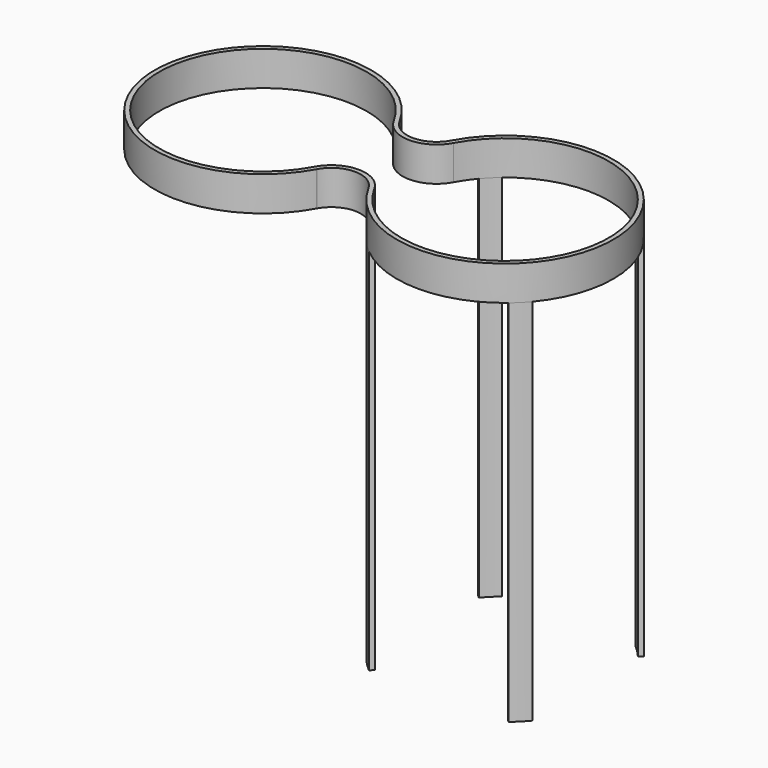
from build123d import *

# Parameters (mm, degrees)
F1_DEPTH = 15
F3_DEPTH = 160


# Not quite as in the source:
# - after a boolean that leaves OpenCascade's solid faulty, fix() repairs it


with BuildPart() as f1:
    # F0 (on Top) → F1 (new body)
    with BuildSketch(Plane.XY):
        with BuildLine():
            ThreePointArc((41.3226906327, -22.3927496943), (52.5, -15.7816452182), (63.6773093673, -22.3927496943))
            ThreePointArc((63.6773093673, -22.3927496943), (63.7058777697, -22.4450182881), (63.7342017495, -22.4974197353))
            ThreePointArc((63.7342017494, -22.4974197352), (152, 0), (63.7342017494, 22.4974197352))
            ThreePointArc((63.7342017494, 22.4974197352), (63.7058777696, 22.445018288), (63.6773093673, 22.3927496943))
            ThreePointArc((63.6773093673, 22.3927496943), (52.5, 15.7816452182), (41.3226906327, 22.3927496943))
            ThreePointArc((41.3226906327, 22.3927496943), (41.2941222304, 22.445018288), (41.2657982506, 22.4974197352))
            ThreePointArc((41.2657982506, 22.4974197352), (-47, 0), (41.2657982506, -22.4974197352))
            ThreePointArc((41.2657982506, -22.4974197352), (41.2941222304, -22.445018288), (41.3226906327, -22.3927496943))
        make_face()
        with BuildLine():
            ThreePointArc((39.5041211148, 21.5505084615), (39.5355894457, 21.4927235868), (39.5669732516, 21.4348927618))
            ThreePointArc((39.5669732516, 21.4348927618), (52.5, 13.7816452182), (65.4330267484, 21.4348927618))
            ThreePointArc((65.4330267484, 21.4348927618), (65.4644105543, 21.4927235868), (65.4958788852, 21.5505084615))
            ThreePointArc((65.4958788852, 21.5505084615), (150, 0), (65.4958788852, -21.5505084615))
            ThreePointArc((65.4958788852, -21.5505084615), (65.4644105543, -21.4927235868), (65.4330267484, -21.4348927618))
            ThreePointArc((65.4330267484, -21.4348927618), (63.4899302841, -18.6916573179), (60.976304449, -16.4594723499))
            ThreePointArc((60.976304449, -16.4594723499), (49.1601952928, -14.1646192224), (39.5669732516, -21.4348927618))
            ThreePointArc((39.5669732516, -21.4348927618), (39.5355894457, -21.4927235868), (39.5041211148, -21.5505084615))
            ThreePointArc((39.5041211148, -21.5505084615), (-45, 0), (39.5041211148, 21.5505084615))
        make_face(mode=Mode.SUBTRACT)
    extrude(amount=F1_DEPTH)

    # F2 (on face) → F3 (join)
    with BuildSketch(Plane(origin=(0, 0, 0), x_dir=(1, 0, 0), z_dir=(0, 0, -1))):
        with BuildLine():
            ThreePointArc((74.7889823447, 36.0040888266), (73.2472602421, 34.6520348301), (71.7659812842, 33.2340187158))
            Line((71.7659812842, 33.2340187158), (73.1801948457, 31.8198051543))
            ThreePointArc((73.1801948466, 31.8198051534), (74.5984406573, 33.1774801565), (76.0745575641, 34.4719999404))
            Line((76.0745575641, 34.4719999404), (74.7889823447, 36.0040888266))
        make_face()
        with BuildLine():
            ThreePointArc((71.7659812842, 33.2340187158), (70.3479651699, 31.7527397579), (68.9959111734, 30.2110176553))
            Line((68.9959111734, 30.2110176553), (70.5280000596, 28.9254424359))
            ThreePointArc((70.5280000596, 28.9254424359), (71.8225198435, 30.4015593427), (73.1801948466, 31.8198051534))
            Line((73.1801948457, 31.8198051543), (71.7659812842, 33.2340187158))
        make_face()
        with BuildLine():
            ThreePointArc((141.0040888266, 30.2110176553), (138.2340187158, 33.2340187158), (135.2110176553, 36.0040888266))
            Line((135.2110176553, 36.0040888266), (133.9254424359, 34.4719999404))
            ThreePointArc((133.9254424359, 34.4719999404), (136.8198051534, 31.8198051534), (139.4719999404, 28.9254424359))
            Line((139.4719999404, 28.9254424359), (141.0040888266, 30.2110176553))
        make_face()
        with BuildLine():
            ThreePointArc((135.2110176553, -36.0040888266), (138.2340187158, -33.2340187158), (141.0040888266, -30.2110176553))
            Line((141.0040888266, -30.2110176553), (139.4719999404, -28.9254424359))
            ThreePointArc((139.4719999404, -28.9254424359), (136.8198051534, -31.8198051534), (133.9254424359, -34.4719999404))
            Line((133.9254424359, -34.4719999404), (135.2110176553, -36.0040888266))
        make_face()
        with BuildLine():
            Line((70.5280000596, -28.9254424359), (68.9959111734, -30.2110176553))
            ThreePointArc((68.9959111734, -30.2110176553), (71.7659812842, -33.2340187158), (74.7889823447, -36.0040888266))
            Line((74.7889823447, -36.0040888266), (76.0745575641, -34.4719999404))
            ThreePointArc((76.0745575641, -34.4719999404), (73.1801948466, -31.8198051534), (70.5280000596, -28.9254424359))
        make_face()
    extrude(amount=F3_DEPTH)

    add(f1.part.fix(), mode=Mode.REPLACE)


solid = f1.part
